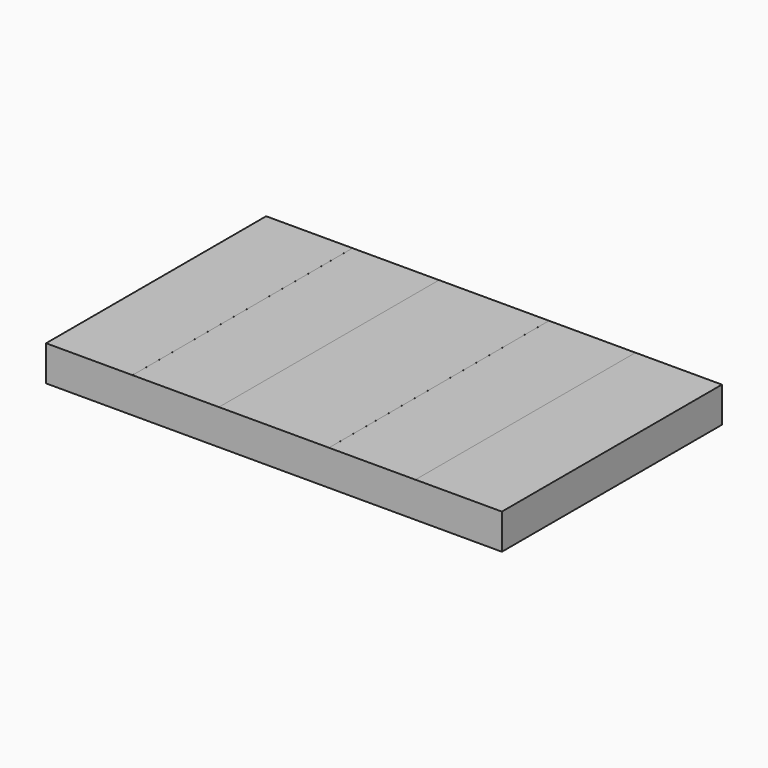
from build123d import *

# Parameters (mm, degrees)
F0_W      = 38.1
F0_H      = 38.1
F1_DEPTH  = 736.6
F2_W      = 38.1
F2_H      = 38.1
F3_DEPTH  = 368.3
F4_W      = 38.1
F4_H      = 38.1
F5_DEPTH  = 736.6
F6_W      = 38.1
F6_H      = 38.1
F7_DEPTH  = 368.3
F8_W      = 101.6
F8_H      = 368.3
F9_DEPTH  = 19.05
F10_W     = 101.6
F10_H     = 368.3
F11_DEPTH = 19.05
F12_W     = 114.3
F12_H     = 368.3
F13_DEPTH = 19.0246
F14_W     = 114.3
F14_H     = 368.3
F15_DEPTH = 19.0246
F16_W     = 177.8
F16_H     = 444.5
F16_W_2   = 152.4
F16_H_2   = 368.3
F17_DEPTH = 19.05


with BuildPart() as f1:
    # F0 (on Right) → F1 (new body)
    with BuildSketch(Plane.YZ):
        with Locations((-19.05, -19.05)):
            Rectangle(F0_W, F0_H)
    extrude(amount=F1_DEPTH)

    # F2 (on face) → F3 (join)
    with BuildSketch(Plane(origin=(0, 0, 0), x_dir=(-1, 0, 0), z_dir=(0, 1, 0))):
        with Locations((-19.05, -19.05)):
            Rectangle(F2_W, F2_H)
        with Locations((-717.55, -19.05)):
            Rectangle(F2_W, F2_H)
    extrude(amount=F3_DEPTH)

    # F4 (on face) → F5 (join)
    with BuildSketch(Plane.YZ.offset(736.6)):
        with Locations((387.35, -19.05)):
            Rectangle(F4_W, F4_H)
    extrude(amount=-F5_DEPTH)

    # F6 (on face) → F7 (join, through all)
    with BuildSketch(Plane.XZ.offset(-368.3)):
        with Locations((273.05, -19.05)):
            Rectangle(F6_W, F6_H)
        with Locations((463.55, -19.05)):
            Rectangle(F6_W, F6_H)
    extrude(amount=F7_DEPTH)

    # F8 (on face) → F9 (join)
    with BuildSketch(Plane.XY):
        Polygon((139.7, 406.4), (0, 406.4), (0, -38.1), (139.7, -38.1), (139.7, 0), (38.1, 0), (38.1, 368.3), (139.7, 368.3), align=None)
        with Locations((88.9, 184.15)):
            Rectangle(F8_W, F8_H)
    extrude(amount=F9_DEPTH)

    # F10 (on face) → F11 (join)
    with BuildSketch(Plane.XY):
        with Locations((647.7, 184.15)):
            Rectangle(F10_W, F10_H)
        Polygon((736.6, -38.1), (736.6, 406.4), (596.9, 406.4), (596.9, 368.3), (698.5, 368.3), (698.5, 0), (596.9, 0), (596.9, -38.1), align=None)
    extrude(amount=F11_DEPTH)

    # F12 (on face) → F13 (join)
    with BuildSketch(Plane.XY):
        Polygon((279.4, 406.4), (139.7, 406.4), (139.7, 368.3), (254, 368.3), (254, 0), (139.7, 0), (139.7, -38.1), (279.4, -38.1), align=None)
        with Locations((196.85, 184.15)):
            Rectangle(F12_W, F12_H)
    extrude(amount=F13_DEPTH)

    # F14 (on face) → F15 (join)
    with BuildSketch(Plane.XY):
        Polygon((596.9, 368.3), (596.9, 406.4), (457.2, 406.4), (457.2, -38.1), (596.9, -38.1), (596.9, 0), (482.6, 0), (482.6, 368.3), align=None)
        with Locations((539.75, 184.15)):
            Rectangle(F14_W, F14_H)
    extrude(amount=F15_DEPTH)

    # F16 (on face) → F17 (join)
    with BuildSketch(Plane.XY):
        with Locations((368.3, 184.15)):
            Rectangle(F16_W, F16_H)
        with Locations((368.3, 184.15)):
            Rectangle(F16_W_2, F16_H_2, mode=Mode.SUBTRACT)
        with Locations((368.3, 184.15)):
            Rectangle(F16_W_2, F16_H_2)
    extrude(amount=F17_DEPTH)


solid = f1.part
